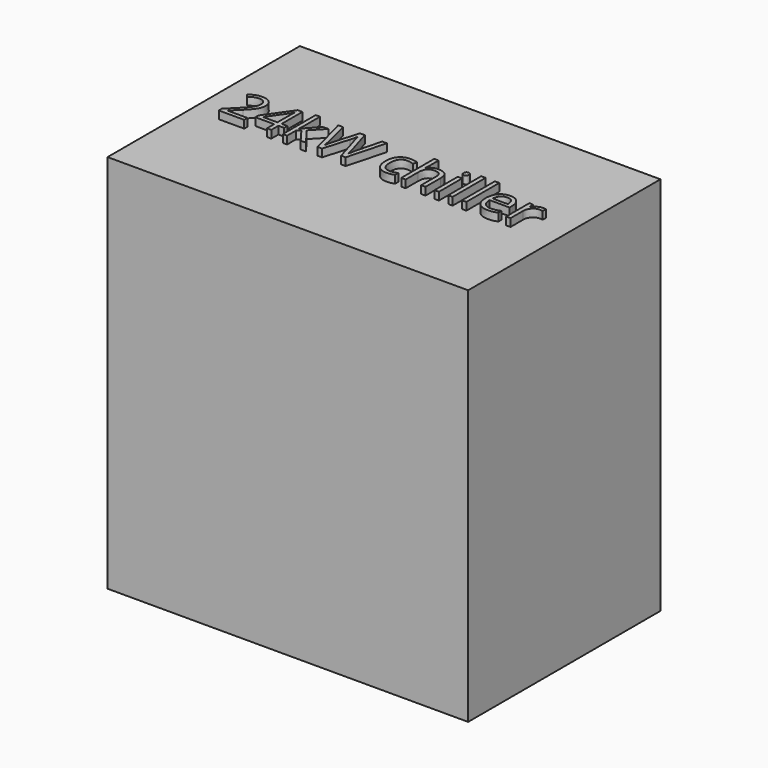
from build123d import *

# Parameters (mm, degrees)
F0_W         = 1181.1
F0_H         = 787.4
F1_DEPTH     = 1244.6
F2_TEXT_SIZE = 177.5399317406
F3_DEPTH     = 25.4


# Not quite as in the source:
# - Text() gives the source's letters only with a copy of the font that has no kerning and outlines rounded to 1/6400 em; it was checked with that copy


with BuildPart() as f1:
    # F0 (on Top) → F1 (new body)
    with BuildSketch(Plane.XY):
        Rectangle(F0_W, F0_H)
    extrude(amount=F1_DEPTH)

    # F2 (on face) → F3 (join)
    with BuildSketch(Plane.XY.offset(1244.6)):
        with Locations((-508, -52.3519761265)):
            Text('24kW chiller', F2_TEXT_SIZE, font='Open Sans', text_align=(TextAlign.LEFT, TextAlign.BOTTOM))
    extrude(amount=F3_DEPTH)


solid = f1.part
